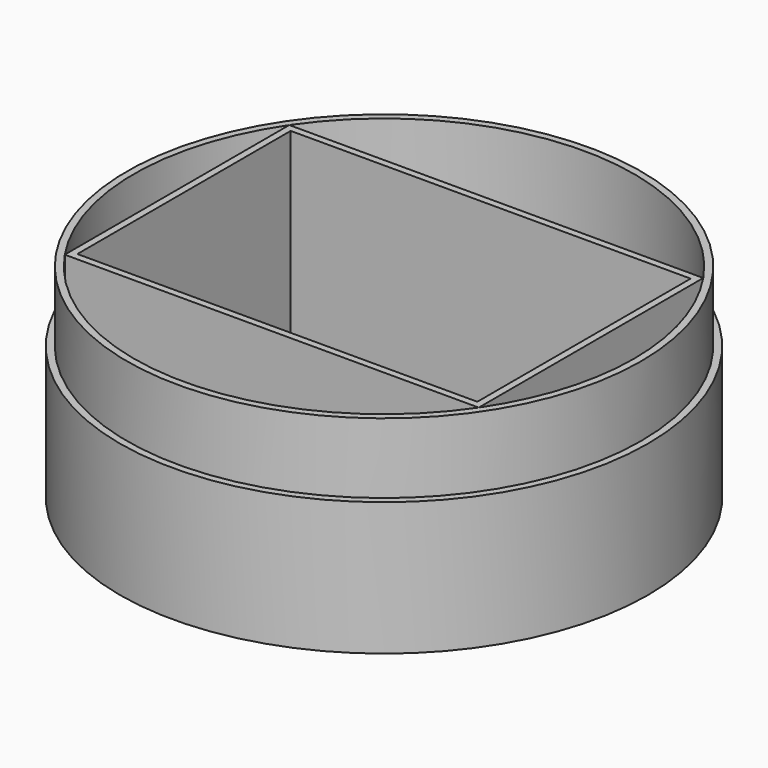
from build123d import *

# Parameters (mm, degrees)
F0_R     = 94.101416936
F1_DEPTH = 72.5
F0_W     = 72.5
F0_H     = 100
F0_W_2   = 2.5
F2_T     = -2.5
F4_DEPTH = 10
F5_R     = 94.101416936
F5_R_2   = 91.601416936
F6_DEPTH = 25


# Not quite as in the source:
# - the program builds the solid bodies; features that only make, move or delete a surface that nothing else refers to are left out


with BuildPart() as f1:
    # F0 (on Top) → F1 (new body)
    with BuildSketch(Plane.XY):
        Circle(F0_R)
        with BuildLine():
            ThreePointArc((89.101416936, 0), (85.177144819, -26.1517972707), (73.75, -50))
            ThreePointArc((73.75, -50), (0, -89.101416936), (-73.75, -50))
            ThreePointArc((-73.75, -50), (-89.101416936, 0), (-73.75, 50))
            ThreePointArc((-73.75, 50), (0, 89.101416936), (73.75, 50))
            ThreePointArc((73.75, 50), (85.177144819, 26.1517972707), (89.101416936, 0))
        make_face(mode=Mode.SUBTRACT)
    extrude(amount=F1_DEPTH)

    # F5 (on face) → F6 (cut)
    with BuildSketch(Plane.XY.offset(72.5)):
        Circle(F5_R)
        Circle(F5_R_2, mode=Mode.SUBTRACT)
    extrude(amount=-F6_DEPTH, mode=Mode.SUBTRACT)


with BuildPart() as f1b:
    # F0 (on Top) → F1, piece 2 (new body)
    with BuildSketch(Plane.XY):
        with Locations((-37.5, 0)):
            Rectangle(F0_W, F0_H)
        with Locations((37.5, 0)):
            Rectangle(F0_W, F0_H)
        Rectangle(F0_W_2, F0_H)
    extrude(amount=F1_DEPTH)

    # F2
    f2_openings = [f1b.faces().sort_by_distance(p)[0] for p in [
        (0, 0, 72.5),
    ]]
    offset(amount=F2_T, openings=f2_openings)


with BuildPart() as f4:
    # F0 (on Top) → F4 (new body)
    with BuildSketch(Plane.XY):
        with BuildLine():
            ThreePointArc((-73.75, 50), (-89.101416936, 0), (-73.75, -50))
            Line((-73.75, -50), (-73.75, 50))
        make_face()
    extrude(amount=F4_DEPTH)


with BuildPart() as f4b:
    # F0 (on Top) → F4, piece 2 (new body)
    with BuildSketch(Plane.XY):
        with BuildLine():
            Line((73.75, 50), (73.75, -50))
            ThreePointArc((73.75, -50), (85.177144819, -26.1517972707), (89.101416936, 0))
            ThreePointArc((89.101416936, 0), (85.177144819, 26.1517972707), (73.75, 50))
        make_face()
    extrude(amount=F4_DEPTH)


with BuildPart() as f4c:
    # F0 (on Top) → F4, piece 3 (new body)
    with BuildSketch(Plane.XY):
        with BuildLine():
            Line((1.25, 50), (73.75, 50))
            ThreePointArc((73.75, 50), (0, 89.101416936), (-73.75, 50))
            Line((-73.75, 50), (-1.25, 50))
            Line((-1.25, 50), (1.25, 50))
        make_face()
    extrude(amount=F4_DEPTH)


with BuildPart() as f4d:
    # F0 (on Top) → F4, piece 4 (new body)
    with BuildSketch(Plane.XY):
        with BuildLine():
            ThreePointArc((-73.75, -50), (0, -89.101416936), (73.75, -50))
            Line((73.75, -50), (1.25, -50))
            Line((1.25, -50), (-1.25, -50))
            Line((-1.25, -50), (-73.75, -50))
        make_face()
    extrude(amount=F4_DEPTH)


solid = Compound([f1.part, f1b.part, f4.part, f4b.part, f4c.part, f4d.part])
